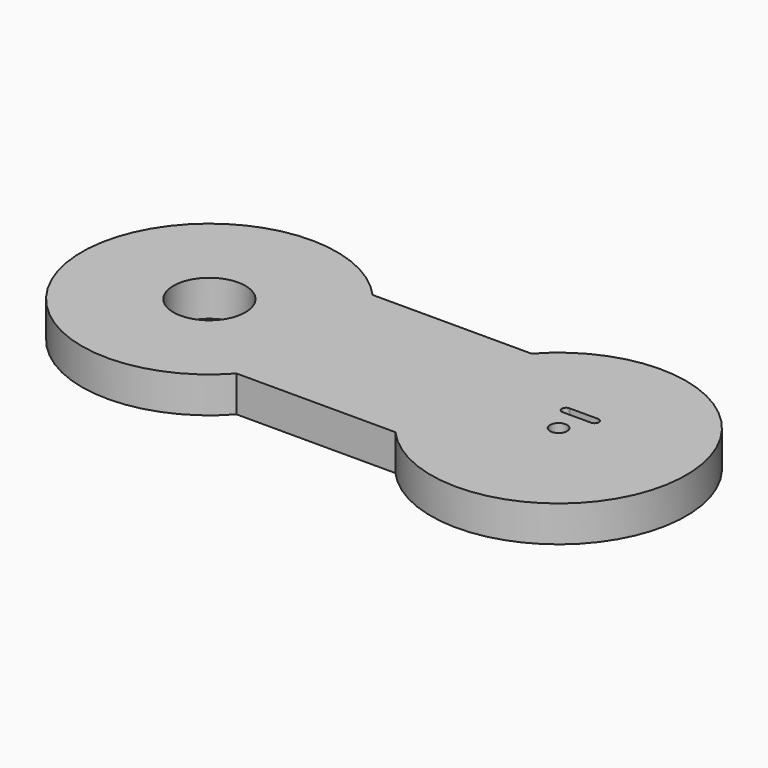
from build123d import *

# Parameters (mm, degrees)
F0_R     = 3
F0_R_2   = 12.7
F1_DEPTH = 12.7


# Not quite as in the source:
# - a feature names something its author has since deleted; it is built from what else it names


with BuildPart() as f1:
    # F0 (on Top) → F1 (new body)
    with BuildSketch(Plane.XY):
        with BuildLine():
            ThreePointArc((56.0618189529, -29.9999992666), (105.6598328516, -42.0377563289), (134.6028392714, 0))
            ThreePointArc((134.6028392714, 0), (105.6598328516, 42.0377563289), (56.0618189529, 29.9999992666))
            ThreePointArc((56.0618189529, 29.9999992666), (44.6028392714, 0), (56.0618189529, -29.9999992666))
        make_face()
        with Locations((89.6028392714, 0)):
            Circle(F0_R, mode=Mode.SUBTRACT)
        with BuildLine():
            ThreePointArc((84.5849392714, 8.08), (83.0886369502, 9.4747414442), (84.3749411096, 11.0652275152))
            ThreePointArc((84.3749411096, 11.0652275152), (84.5827763317, 11.0799984406), (84.7906532876, 11.0658269561))
            Line((84.7906532876, 11.0658269561), (94.6185763317, 11.0799984406))
            ThreePointArc((94.6185763317, 11.0799984406), (95.6806344526, 10.641424611), (96.1207392714, 9.58))
            ThreePointArc((96.1207392714, 9.58), (95.6813994432, 8.5193398282), (94.6207392714, 8.08))
            Line((94.6207392714, 8.08), (84.5849392714, 8.08))
        make_face(mode=Mode.SUBTRACT)
        with BuildLine():
            ThreePointArc((56.0618189529, -29.9999992666), (44.6028392714, 0), (56.0618189529, 29.9999992666))
            Line((56.0618189529, 29.9999992666), (0, 29.9999992666))
            ThreePointArc((0, 29.9999992666), (8.4967360104, 16.0569935802), (11.4589796815, 0))
            ThreePointArc((11.4589796815, 0), (8.4967360104, -16.0569935802), (0, -29.9999992666))
            Line((0, -29.9999992666), (56.0618189529, -29.9999992666))
        make_face()
        with BuildLine():
            ThreePointArc((11.4589796815, 0), (8.4967360104, 16.0569935802), (0, 29.9999992666))
            ThreePointArc((0, 29.9999992666), (-78.5410203185, 0), (0, -29.9999992666))
            ThreePointArc((0, -29.9999992666), (8.4967360104, -16.0569935802), (11.4589796815, 0))
        make_face()
        with Locations((-33.5410203185, 0)):
            Circle(F0_R_2, mode=Mode.SUBTRACT)
    extrude(amount=F1_DEPTH)


solid = f1.part
